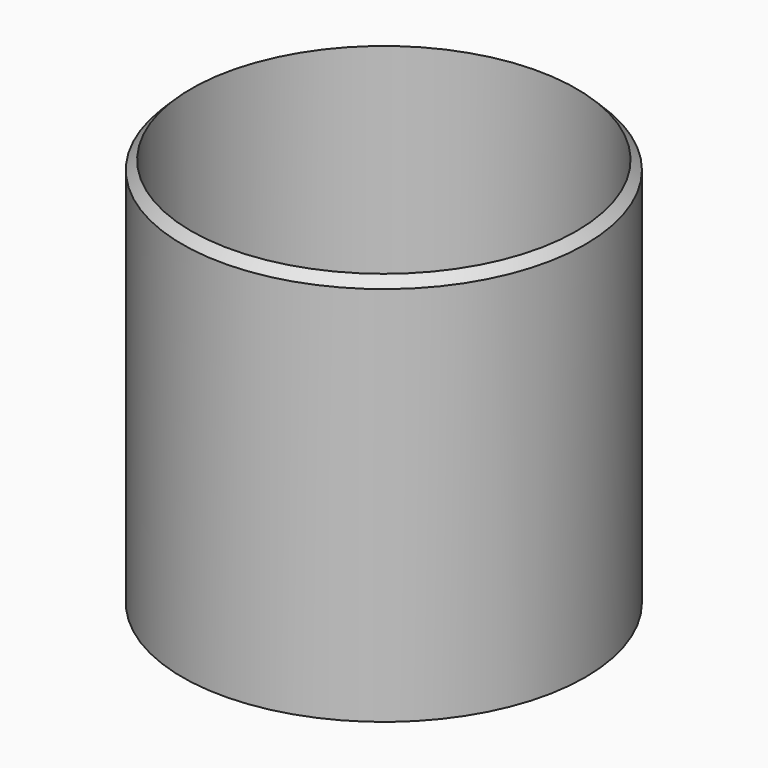
from build123d import *

# Parameters (mm, degrees)
F0_R     = 57.7707410697
F1_DEPTH = 114.3
F2_T     = -2.54


# Not quite as in the source:
# - a fillet or chamfer that OpenCascade refuses, or shapes differently, is made with other operations: its cross-section is extruded or revolved along the edge and cut away or added
# - the program builds the solid bodies; features that only make, move or delete a surface that nothing else refers to are left out


with BuildPart() as f1:
    # F0 (on Top) → F1 (new body)
    with BuildSketch(Plane.XY):
        Circle(F0_R)
    extrude(amount=-F1_DEPTH)

    # F2
    f2_openings = [f1.faces().sort_by_distance(p)[0] for p in [
        (0, 0, 0),
    ]]
    offset(amount=F2_T, openings=f2_openings)

    # F3: chamfer of 5.08 on 1 edges, made by hand

    # F3_s1 → F3_t2 (revolve, cut)
    with BuildSketch(Plane.XZ):
        Polygon((57.7707410697, -5.08), (52.6907410697, 0), (57.7707410697, 0), align=None)
    revolve(axis=Axis((0, 0, 0), (0, 0, 1)), mode=Mode.SUBTRACT)


solid = f1.part
